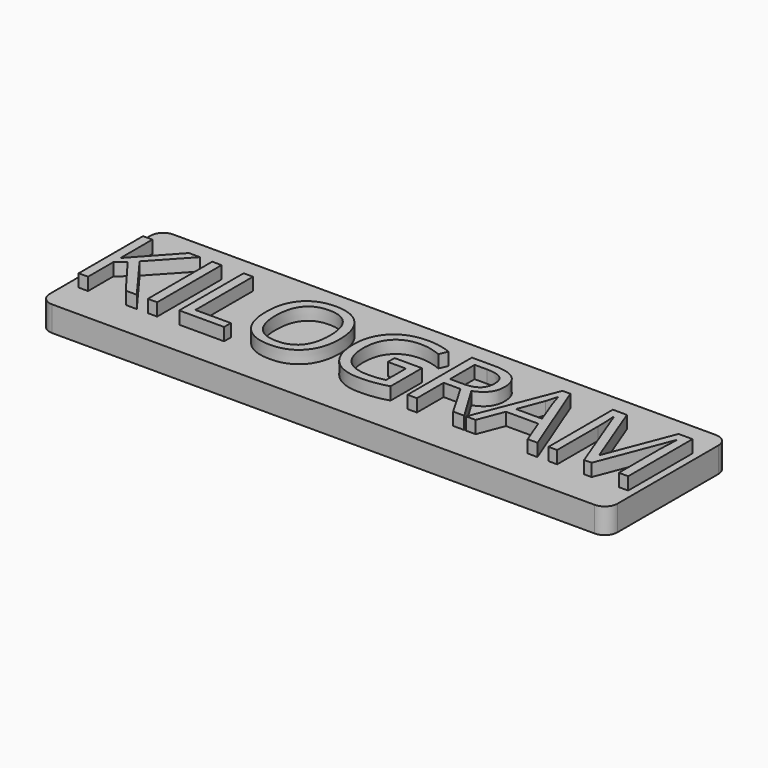
from build123d import *

# Parameters (mm, degrees)
F0_W         = 90
F0_H         = 24
F1_DEPTH     = 4
F2_R         = 2
F3_TEXT_SIZE = 17.8599113206
F4_DEPTH     = 2
F5_TEXT_SIZE = 17.3611111111
F6_DEPTH     = 1.5


# Not quite as in the source:
# - a feature names something its author has since deleted; it is built from what else it names
# - Text() gives the source's letters only with a copy of the font that has no kerning and outlines rounded to 1/6400 em; it was checked with that copy


with BuildPart() as f1:
    # F0 (on Top) → F1 (new body)
    with BuildSketch(Plane.XY):
        Rectangle(F0_W, F0_H)
    extrude(amount=F1_DEPTH)

    # F2
    f2_edges = [f1.edges().sort_by_distance(p)[0] for p in [
        (-45, -12, 2),
        (45, 12, 2),
        (-45, 12, 2),
        (45, -12, 2),
    ]]
    fillet(f2_edges, radius=F2_R)

    # F3 (on face) → F4 (join)
    with BuildSketch(Plane.XY.offset(4)):
        with Locations((-45, -6.4295680754)):
            Text('KILOGRAM', F3_TEXT_SIZE, font='Open Sans', text_align=(TextAlign.LEFT, TextAlign.BOTTOM))
    extrude(amount=F4_DEPTH)

    # F5 (on face) → F6 (cut)
    with BuildSketch(Plane(origin=(0, 0, 0), x_dir=(1, 0, 0), z_dir=(0, 0, -1))):
        with Locations((-26.311577691, -6.25)):
            Text('2.2 lbs', F5_TEXT_SIZE, font='Open Sans', text_align=(TextAlign.LEFT, TextAlign.BOTTOM))
    extrude(amount=-F6_DEPTH, mode=Mode.SUBTRACT)


solid = f1.part
